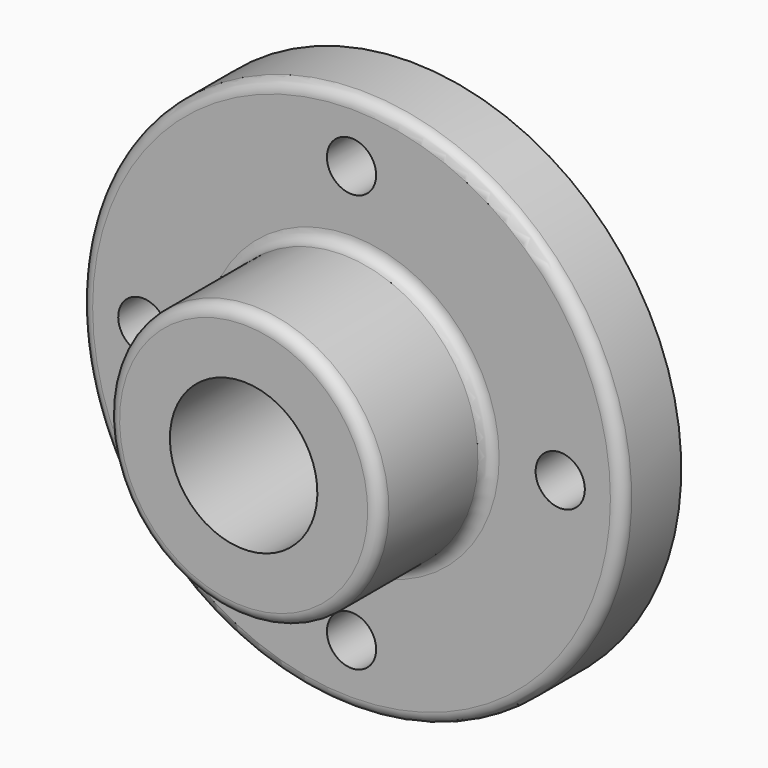
from build123d import *

# Parameters (mm, degrees)
F2_R            = 3.048
F3_R            = 6.35
F4_DEPTH        = 19.051
F4_COPIES_COUNT = 4


# Not quite as in the source:
# - a pattern or mirror of a feature is missing from the dataset's text; its kind, count and spacing are read off the source's solid


with BuildPart() as f1:
    # F0 (on Right) → F1 (revolve)
    with BuildSketch(Plane.YZ):
        Polygon((-26.924, 35.052), (-26.924, 19.0246), (26.924, 19.0246), (26.924, 69.85), (7.874, 69.85), (7.874, 35.052), align=None)
    revolve(axis=Axis((0, 0, 0), (0, 1, 0)))

    # F2
    f2_edges = [f1.edges().sort_by_distance(p)[0] for p in [
        (0, -26.924, -35.052),
        (0, 7.874, -69.85),
        (0, 7.874, -35.052),
    ]]
    fillet(f2_edges, radius=F2_R)

    # F3 (on face) → F4 (cut, through all)
    with BuildSketch(Plane.XZ.offset(-7.874)):
        with Locations((0, 53.848)):
            Circle(F3_R)
    f4 = extrude(amount=-F4_DEPTH, mode=Mode.SUBTRACT)

    # F4_copies: F4 ×4 about axis
    f4_copies_axis = Axis((0, 0, 0), (0, 1, 0))
    for i in range(1, F4_COPIES_COUNT):
        add(f4.rotate(f4_copies_axis, i * 360 / F4_COPIES_COUNT), mode=Mode.SUBTRACT)


solid = f1.part
